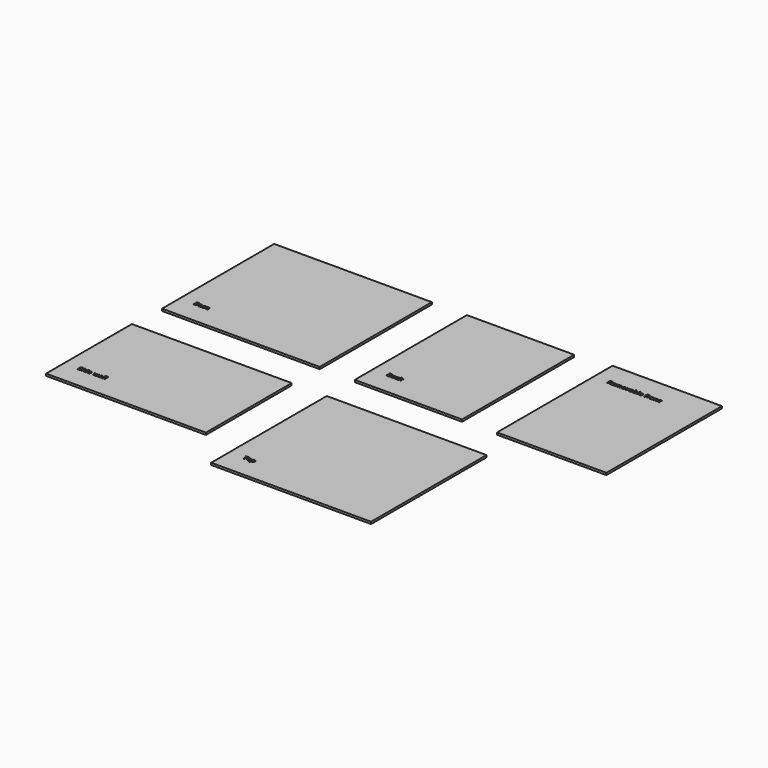
from build123d import *

# Parameters (mm, degrees)
F0_W     = 450
F0_H     = 400
F1_DEPTH = 6
F0_W_2   = 306
F2_DEPTH = 6
F0_W_3   = 456
F0_H_2   = 306
F0_W_4   = 2.7071983507
F0_H_3   = 9.9254470486
F0_H_4   = 13.8143815104
F3_DEPTH = 6
F0_H_5   = 412
F4_DEPTH = 6
F0_W_5   = 312
F5_DEPTH = 6


with BuildPart() as f1:
    # F0 (on Top) → F1 (new body)
    with BuildSketch(Plane.XY):
        with Locations((-275, 250)):
            Rectangle(F0_W, F0_H)
        with BuildLine():
            Line((-438.1719704861, 110), (-440.0610438368, 110))
            Line((-440.0610438368, 110), (-440.5865755208, 111.3493381076))
            Line((-440.5865755208, 111.3493381076), (-440.657593316, 111.3493381076))
            add(Edge.make_bspline(
                [(-440.657593316, 111.3493381076), (-441.3393641493, 110.4886024306), (-442.0637456597, 110.1548187934)],
                knots=[0, 0, 0, 1, 1, 1], degree=2))
            add(Edge.make_bspline(
                [(-442.0637456597, 110.1548187934), (-442.7881271701, 109.8210351562), (-443.9499782986, 109.8210351562)],
                knots=[0, 0, 0, 1, 1, 1], degree=2))
            add(Edge.make_bspline(
                [(-443.9499782986, 109.8210351562), (-445.3788563368, 109.8210351562), (-446.1998220486, 110.6391601562)],
                knots=[0, 0, 0, 1, 1, 1], degree=2))
            add(Edge.make_bspline(
                [(-446.1998220486, 110.6391601562), (-447.0207877604, 111.4572851562), (-447.0207877604, 112.965703125)],
                knots=[0, 0, 0, 1, 1, 1], degree=2))
            add(Edge.make_bspline(
                [(-447.0207877604, 112.965703125), (-447.0207877604, 114.5451388889), (-445.9157508681, 115.2950868056)],
                knots=[0, 0, 0, 1, 1, 1], degree=2))
            add(Edge.make_bspline(
                [(-445.9157508681, 115.2950868056), (-444.8107139757, 116.0450347222), (-442.5835959201, 116.1245746528)],
                knots=[0, 0, 0, 1, 1, 1], degree=2))
            Line((-442.5835959201, 116.1245746528), (-440.8592838542, 116.1785481771))
            Line((-440.8592838542, 116.1785481771), (-440.8592838542, 116.6131770833))
            add(Edge.make_bspline(
                [(-440.8592838542, 116.6131770833), (-440.8592838542, 118.1215950521), (-442.4046310764, 118.1215950521)],
                knots=[0, 0, 0, 1, 1, 1], degree=2))
            add(Edge.make_bspline(
                [(-442.4046310764, 118.1215950521), (-443.5948893229, 118.1215950521), (-445.2027322049, 117.4028949653)],
                knots=[0, 0, 0, 1, 1, 1], degree=2))
            Line((-445.2027322049, 117.4028949653), (-446.0975564236, 119.2323133681))
            add(Edge.make_bspline(
                [(-446.0975564236, 119.2323133681), (-444.3846072049, 120.1299782986), (-442.2995247396, 120.1299782986)],
                knots=[0, 0, 0, 1, 1, 1], degree=2))
            add(Edge.make_bspline(
                [(-442.2995247396, 120.1299782986), (-440.3025043403, 120.1299782986), (-439.2372374132, 119.2593001302)],
                knots=[0, 0, 0, 1, 1, 1], degree=2))
            add(Edge.make_bspline(
                [(-439.2372374132, 119.2593001302), (-438.1719704861, 118.3886219618), (-438.1719704861, 116.6131770833)],
                knots=[0, 0, 0, 1, 1, 1], degree=2))
            Line((-438.1719704861, 116.6131770833), (-438.1719704861, 110))
        make_face(mode=Mode.SUBTRACT)
        with BuildLine():
            add(Edge.make_bspline(
                [(-428.7152408854, 114.2170366753), (-428.4567361111, 113.6844032118), (-428.4567361111, 112.9486588542)],
                knots=[0, 0, 0, 1, 1, 1], degree=2))
            add(Edge.make_bspline(
                [(-428.4567361111, 112.9486588542), (-428.4567361111, 111.4203559028), (-429.5177419705, 110.6206955295)],
                knots=[0, 0, 0, 1, 1, 1], degree=2))
            add(Edge.make_bspline(
                [(-429.5177419705, 110.6206955295), (-430.5787478299, 109.8210351562), (-432.6922374132, 109.8210351562)],
                knots=[0, 0, 0, 1, 1, 1], degree=2))
            add(Edge.make_bspline(
                [(-432.6922374132, 109.8210351562), (-433.7745486111, 109.8210351562), (-434.5387000868, 109.9687521701)],
                knots=[0, 0, 0, 1, 1, 1], degree=2))
            add(Edge.make_bspline(
                [(-434.5387000868, 109.9687521701), (-435.3028515625, 110.116469184), (-435.967578125, 110.4005403646)],
                knots=[0, 0, 0, 1, 1, 1], degree=2))
            Line((-435.967578125, 110.4005403646), (-435.967578125, 112.6361805556))
            add(Edge.make_bspline(
                [(-435.967578125, 112.6361805556), (-435.2147894965, 112.2810915799), (-434.2688324653, 112.0410514323)],
                knots=[0, 0, 0, 1, 1, 1], degree=2))
            add(Edge.make_bspline(
                [(-434.2688324653, 112.0410514323), (-433.322875434, 111.8010112847), (-432.6041753472, 111.8010112847)],
                knots=[0, 0, 0, 1, 1, 1], degree=2))
            add(Edge.make_bspline(
                [(-432.6041753472, 111.8010112847), (-431.1298459201, 111.8010112847), (-431.1298459201, 112.6532248264)],
                knots=[0, 0, 0, 1, 1, 1], degree=2))
            add(Edge.make_bspline(
                [(-431.1298459201, 112.6532248264), (-431.1298459201, 112.9742252604), (-431.3258550347, 113.1744954427)],
                knots=[0, 0, 0, 1, 1, 1], degree=2))
            add(Edge.make_bspline(
                [(-431.3258550347, 113.1744954427), (-431.5218641493, 113.374765625), (-432.0005240885, 113.6275889757)],
                knots=[0, 0, 0, 1, 1, 1], degree=2))
            add(Edge.make_bspline(
                [(-432.0005240885, 113.6275889757), (-432.4791840278, 113.8804123264), (-433.2774240451, 114.2156163194)],
                knots=[0, 0, 0, 1, 1, 1], degree=2))
            add(Edge.make_bspline(
                [(-433.2774240451, 114.2156163194), (-434.4222309028, 114.6956966146), (-434.9605457899, 115.1047591146)],
                knots=[0, 0, 0, 1, 1, 1], degree=2))
            add(Edge.make_bspline(
                [(-434.9605457899, 115.1047591146), (-435.4988606771, 115.5138216146), (-435.7417415365, 116.0421940104)],
                knots=[0, 0, 0, 1, 1, 1], degree=2))
            add(Edge.make_bspline(
                [(-435.7417415365, 116.0421940104), (-435.9846223958, 116.5705664062), (-435.9846223958, 117.3403993056)],
                knots=[0, 0, 0, 1, 1, 1], degree=2))
            add(Edge.make_bspline(
                [(-435.9846223958, 117.3403993056), (-435.9846223958, 118.6641710069), (-434.9605457899, 119.3871321615)],
                knots=[0, 0, 0, 1, 1, 1], degree=2))
            add(Edge.make_bspline(
                [(-434.9605457899, 119.3871321615), (-433.936469184, 120.110093316), (-432.0530772569, 120.110093316)],
                knots=[0, 0, 0, 1, 1, 1], degree=2))
            add(Edge.make_bspline(
                [(-432.0530772569, 120.110093316), (-430.2605881076, 120.110093316), (-428.5646831597, 119.3288975694)],
                knots=[0, 0, 0, 1, 1, 1], degree=2))
            Line((-428.5646831597, 119.3288975694), (-429.3799674479, 117.377328559))
            add(Edge.make_bspline(
                [(-429.3799674479, 117.377328559), (-430.1270746528, 117.6954882812), (-430.7747569444, 117.9000195312)],
                knots=[0, 0, 0, 1, 1, 1], degree=2))
            add(Edge.make_bspline(
                [(-430.7747569444, 117.9000195312), (-431.4224392361, 118.1045507812), (-432.0985286458, 118.1045507812)],
                knots=[0, 0, 0, 1, 1, 1], degree=2))
            add(Edge.make_bspline(
                [(-432.0985286458, 118.1045507812), (-433.2973090278, 118.1045507812), (-433.2973090278, 117.4568684896)],
                knots=[0, 0, 0, 1, 1, 1], degree=2))
            add(Edge.make_bspline(
                [(-433.2973090278, 117.4568684896), (-433.2973090278, 117.0932573785), (-432.9109722222, 116.8262304687)],
                knots=[0, 0, 0, 1, 1, 1], degree=2))
            add(Edge.make_bspline(
                [(-432.9109722222, 116.8262304687), (-432.5246354167, 116.559203559), (-431.2179079861, 116.0365125868)],
                knots=[0, 0, 0, 1, 1, 1], degree=2))
            add(Edge.make_bspline(
                [(-431.2179079861, 116.0365125868), (-430.0560568576, 115.5649544271), (-429.5149012587, 115.157312283)],
                knots=[0, 0, 0, 1, 1, 1], degree=2))
            add(Edge.make_bspline(
                [(-429.5149012587, 115.157312283), (-428.9737456597, 114.7496701389), (-428.7152408854, 114.2170366753)],
                knots=[0, 0, 0, 1, 1, 1], degree=2))
        make_face(mode=Mode.SUBTRACT)
        with BuildLine():
            add(Edge.make_bspline(
                [(-419.8834678819, 109.9943185764), (-420.6902300347, 109.8210351562), (-421.854921875, 109.8210351562)],
                knots=[0, 0, 0, 1, 1, 1], degree=2))
            add(Edge.make_bspline(
                [(-421.854921875, 109.8210351562), (-424.2496419271, 109.8210351562), (-425.5989800347, 111.1448068576)],
                knots=[0, 0, 0, 1, 1, 1], degree=2))
            add(Edge.make_bspline(
                [(-425.5989800347, 111.1448068576), (-426.9483181424, 112.468578559), (-426.9483181424, 114.8917057292)],
                knots=[0, 0, 0, 1, 1, 1], degree=2))
            add(Edge.make_bspline(
                [(-426.9483181424, 114.8917057292), (-426.9483181424, 117.3858506944), (-425.7012456597, 118.7479720052)],
                knots=[0, 0, 0, 1, 1, 1], degree=2))
            add(Edge.make_bspline(
                [(-425.7012456597, 118.7479720052), (-424.4541731771, 120.110093316), (-422.2526215278, 120.110093316)],
                knots=[0, 0, 0, 1, 1, 1], degree=2))
            add(Edge.make_bspline(
                [(-422.2526215278, 120.110093316), (-420.1504947917, 120.110093316), (-418.9787011719, 118.9127332899)],
                knots=[0, 0, 0, 1, 1, 1], degree=2))
            add(Edge.make_bspline(
                [(-418.9787011719, 118.9127332899), (-417.8069075521, 117.7153732639), (-417.8069075521, 115.6018836806)],
                knots=[0, 0, 0, 1, 1, 1], degree=2))
            Line((-417.8069075521, 115.6018836806), (-417.8069075521, 114.2866341146))
            Line((-417.8069075521, 114.2866341146), (-424.20703125, 114.2866341146))
            add(Edge.make_bspline(
                [(-424.20703125, 114.2866341146), (-424.1615798611, 113.1333051215), (-423.5224197049, 112.4856228299)],
                knots=[0, 0, 0, 1, 1, 1], degree=2))
            add(Edge.make_bspline(
                [(-423.5224197049, 112.4856228299), (-422.8832595486, 111.8379405382), (-421.7299305556, 111.8379405382)],
                knots=[0, 0, 0, 1, 1, 1], degree=2))
            add(Edge.make_bspline(
                [(-421.7299305556, 111.8379405382), (-420.832265625, 111.8379405382), (-420.0340256076, 112.0240071615)],
                knots=[0, 0, 0, 1, 1, 1], degree=2))
            add(Edge.make_bspline(
                [(-420.0340256076, 112.0240071615), (-419.2357855903, 112.2100737847), (-418.3665277778, 112.6191362847)],
                knots=[0, 0, 0, 1, 1, 1], degree=2))
            Line((-418.3665277778, 112.6191362847), (-418.3665277778, 110.5226909722))
            add(Edge.make_bspline(
                [(-418.3665277778, 110.5226909722), (-419.0767057292, 110.1676019965), (-419.8834678819, 109.9943185764)],
                knots=[0, 0, 0, 1, 1, 1], degree=2))
        make_face(mode=Mode.SUBTRACT)
        with BuildLine():
            Line((-458.3665907118, 110), (-458.3665907118, 122.9792122396))
            Line((-458.3665907118, 122.9792122396), (-454.3270985243, 122.9792122396))
            add(Edge.make_bspline(
                [(-454.3270985243, 122.9792122396), (-451.5659266493, 122.9792122396), (-450.3188541667, 122.1937554253)],
                knots=[0, 0, 0, 1, 1, 1], degree=2))
            add(Edge.make_bspline(
                [(-450.3188541667, 122.1937554253), (-449.071781684, 121.4082986111), (-449.071781684, 119.6953493924)],
                knots=[0, 0, 0, 1, 1, 1], degree=2))
            add(Edge.make_bspline(
                [(-449.071781684, 119.6953493924), (-449.071781684, 118.5306575521), (-449.6171983507, 117.7849707031)],
                knots=[0, 0, 0, 1, 1, 1], degree=2))
            add(Edge.make_bspline(
                [(-449.6171983507, 117.7849707031), (-450.1626150174, 117.0392838542), (-451.0688020833, 116.8887261285)],
                knots=[0, 0, 0, 1, 1, 1], degree=2))
            Line((-451.0688020833, 116.8887261285), (-451.0688020833, 116.8006640625))
            add(Edge.make_bspline(
                [(-451.0688020833, 116.8006640625), (-449.8359331597, 116.5251150174), (-449.2890961372, 115.770906033)],
                knots=[0, 0, 0, 1, 1, 1], degree=2))
            add(Edge.make_bspline(
                [(-449.2890961372, 115.770906033), (-448.7422591146, 115.0166970486), (-448.7422591146, 113.7639431424)],
                knots=[0, 0, 0, 1, 1, 1], degree=2))
            add(Edge.make_bspline(
                [(-448.7422591146, 113.7639431424), (-448.7422591146, 111.9884982639), (-450.0262608507, 110.9942491319)],
                knots=[0, 0, 0, 1, 1, 1], degree=2))
            add(Edge.make_bspline(
                [(-450.0262608507, 110.9942491319), (-451.3102625868, 110), (-453.5118142361, 110)],
                knots=[0, 0, 0, 1, 1, 1], degree=2))
            Line((-453.5118142361, 110), (-458.3665907118, 110))
        make_face(mode=Mode.SUBTRACT)
    extrude(amount=F1_DEPTH)


with BuildPart() as f2:
    # F0 (on Top) → F2 (new body)
    with BuildSketch(Plane.XY):
        with Locations((203, 250)):
            Rectangle(F0_W_2, F0_H)
        with BuildLine():
            Line((111.8281674137, 110), (109.9390821287, 110))
            Line((109.9390821287, 110), (109.4135471246, 111.3493466322))
            Line((109.4135471246, 111.3493466322), (109.3425288808, 111.3493466322))
            add(Edge.make_bspline(
                [(109.3425288808, 111.3493466322), (108.6607537403, 110.4886055173), (107.9363676536, 110.1548197715)],
                knots=[0, 0, 0, 1, 1, 1], degree=2))
            add(Edge.make_bspline(
                [(107.9363676536, 110.1548197715), (107.2119815668, 109.8210340256), (106.0501230983, 109.8210340256)],
                knots=[0, 0, 0, 1, 1, 1], degree=2))
            add(Edge.make_bspline(
                [(106.0501230983, 109.8210340256), (104.6212360331, 109.8210340256), (103.8002651348, 110.6391641942)],
                knots=[0, 0, 0, 1, 1, 1], degree=2))
            add(Edge.make_bspline(
                [(103.8002651348, 110.6391641942), (102.9792942365, 111.4572943627), (102.9792942365, 112.965721861)],
                knots=[0, 0, 0, 1, 1, 1], degree=2))
            add(Edge.make_bspline(
                [(102.9792942365, 112.965721861), (102.9792942365, 114.5451676031), (104.08433811, 115.2951202576)],
                knots=[0, 0, 0, 1, 1, 1], degree=2))
            add(Edge.make_bspline(
                [(104.08433811, 115.2951202576), (105.1893819835, 116.0450729121), (107.416514109, 116.1246133451)],
                knots=[0, 0, 0, 1, 1, 1], degree=2))
            Line((107.416514109, 116.1246133451), (109.1408370684, 116.1785872104))
            Line((109.1408370684, 116.1785872104), (109.1408370684, 116.6132188624))
            add(Edge.make_bspline(
                [(109.1408370684, 116.6132188624), (109.1408370684, 118.1216463607), (107.5954800833, 118.1216463607)],
                knots=[0, 0, 0, 1, 1, 1], degree=2))
            add(Edge.make_bspline(
                [(107.5954800833, 118.1216463607), (106.4052143173, 118.1216463607), (104.7973612777, 117.4029417335)],
                knots=[0, 0, 0, 1, 1, 1], degree=2))
            Line((104.7973612777, 117.4029417335), (103.9025314058, 119.2323716937))
            add(Edge.make_bspline(
                [(103.9025314058, 119.2323716937), (105.6154914462, 120.1300422953), (107.7005870841, 120.1300422953)],
                knots=[0, 0, 0, 1, 1, 1], degree=2))
            add(Edge.make_bspline(
                [(107.7005870841, 120.1300422953), (109.6976200997, 120.1300422953), (110.7628937567, 119.2593586263)],
                knots=[0, 0, 0, 1, 1, 1], degree=2))
            add(Edge.make_bspline(
                [(110.7628937567, 119.2593586263), (111.8281674137, 118.3886749574), (111.8281674137, 116.6132188624)],
                knots=[0, 0, 0, 1, 1, 1], degree=2))
            Line((111.8281674137, 116.6132188624), (111.8281674137, 110))
        make_face(mode=Mode.SUBTRACT)
        with BuildLine():
            add(Edge.make_bspline(
                [(120.3389937504, 109.9815352566), (119.6685815289, 109.8210340256), (118.648759548, 109.8210340256)],
                knots=[0, 0, 0, 1, 1, 1], degree=2))
            add(Edge.make_bspline(
                [(118.648759548, 109.8210340256), (114.0155293226, 109.8210340256), (114.0155293226, 114.9087810113)],
                knots=[0, 0, 0, 1, 1, 1], degree=2))
            add(Edge.make_bspline(
                [(114.0155293226, 114.9087810113), (114.0155293226, 117.4398712203), (115.2753929676, 118.7750142036)],
                knots=[0, 0, 0, 1, 1, 1], degree=2))
            add(Edge.make_bspline(
                [(115.2753929676, 118.7750142036), (116.5352566126, 120.110157187), (118.8873808472, 120.110157187)],
                knots=[0, 0, 0, 1, 1, 1], degree=2))
            add(Edge.make_bspline(
                [(118.8873808472, 120.110157187), (120.6088630768, 120.110157187), (121.9780948172, 119.4369042358)],
                knots=[0, 0, 0, 1, 1, 1], degree=2))
            Line((121.9780948172, 119.4369042358), (121.1770090272, 117.3404456789))
            add(Edge.make_bspline(
                [(121.1770090272, 117.3404456789), (120.537844833, 117.5989520864), (119.988163626, 117.763714412)],
                knots=[0, 0, 0, 1, 1, 1], degree=2))
            add(Edge.make_bspline(
                [(119.988163626, 117.763714412), (119.438482419, 117.9284767376), (118.8873808472, 117.9284767376)],
                knots=[0, 0, 0, 1, 1, 1], degree=2))
            add(Edge.make_bspline(
                [(118.8873808472, 117.9284767376), (116.7738779117, 117.9284767376), (116.7738779117, 114.9258253898)],
                knots=[0, 0, 0, 1, 1, 1], degree=2))
            add(Edge.make_bspline(
                [(116.7738779117, 114.9258253898), (116.7738779117, 112.0140773941), (118.8873808472, 112.0140773941)],
                knots=[0, 0, 0, 1, 1, 1], degree=2))
            add(Edge.make_bspline(
                [(118.8873808472, 112.0140773941), (119.6685815289, 112.0140773941), (120.3347326558, 112.2228710309)],
                knots=[0, 0, 0, 1, 1, 1], degree=2))
            add(Edge.make_bspline(
                [(120.3347326558, 112.2228710309), (121.0008837826, 112.4316646676), (121.6656145445, 112.8776592387)],
                knots=[0, 0, 0, 1, 1, 1], degree=2))
            Line((121.6656145445, 112.8776592387), (121.6656145445, 110.5596237611))
            add(Edge.make_bspline(
                [(121.6656145445, 110.5596237611), (121.0094059718, 110.1420364876), (120.3389937504, 109.9815352566)],
                knots=[0, 0, 0, 1, 1, 1], degree=2))
        make_face(mode=Mode.SUBTRACT)
        with BuildLine():
            Line((91.6334196073, 110), (91.6334196073, 122.9792942365))
            Line((91.6334196073, 122.9792942365), (95.6729373146, 122.9792942365))
            add(Edge.make_bspline(
                [(95.6729373146, 122.9792942365), (98.4341266334, 122.9792942365), (99.6812069945, 122.1938324601)],
                knots=[0, 0, 0, 1, 1, 1], degree=2))
            add(Edge.make_bspline(
                [(99.6812069945, 122.1938324601), (100.9282873556, 121.4083706837), (100.9282873556, 119.6954106433)],
                knots=[0, 0, 0, 1, 1, 1], degree=2))
            add(Edge.make_bspline(
                [(100.9282873556, 119.6954106433), (100.9282873556, 118.530711445), (100.3828672432, 117.7850198851)],
                knots=[0, 0, 0, 1, 1, 1], degree=2))
            add(Edge.make_bspline(
                [(100.3828672432, 117.7850198851), (99.8374471309, 117.0393283252), (98.93125434, 116.8887696484)],
                knots=[0, 0, 0, 1, 1, 1], degree=2))
            Line((98.93125434, 116.8887696484), (98.93125434, 116.8007070261))
            add(Edge.make_bspline(
                [(98.93125434, 116.8007070261), (100.1641310523, 116.5251562401), (100.7109715296, 115.770942491)],
                knots=[0, 0, 0, 1, 1, 1], degree=2))
            add(Edge.make_bspline(
                [(100.7109715296, 115.770942491), (101.2578120068, 115.0167287419), (101.2578120068, 113.7639669213)],
                knots=[0, 0, 0, 1, 1, 1], degree=2))
            add(Edge.make_bspline(
                [(101.2578120068, 113.7639669213), (101.2578120068, 111.9885108263), (99.973802159, 110.9942554132)],
                knots=[0, 0, 0, 1, 1, 1], degree=2))
            add(Edge.make_bspline(
                [(99.973802159, 110.9942554132), (98.6897923111, 110), (96.4882267534, 110)],
                knots=[0, 0, 0, 1, 1, 1], degree=2))
            Line((96.4882267534, 110), (91.6334196073, 110))
        make_face(mode=Mode.SUBTRACT)
        Polygon((126.5317846096, 115.3973865286), (126.5687140963, 115.3973865286), (127.7476169434, 116.9058140269), (130.5258506407, 119.9255097532), (133.579635124, 119.9255097532), (129.6395429581, 115.6189634493), (133.821097153, 110), (130.6962944259, 110), (127.8385202954, 114.0224733287), (126.6738210972, 113.0907139701), (126.6738210972, 110), (123.9666056436, 110), (123.9666056436, 123.8144687835), (126.6738210972, 123.8144687835), (126.6738210972, 117.6529259516), align=None, mode=Mode.SUBTRACT)
    extrude(amount=F2_DEPTH)


with BuildPart() as f3:
    # F0 (on Top) → F3 (new body)
    with BuildSketch(Plane.XY):
        with Locations((-278, -203)):
            Rectangle(F0_W_3, F0_H_2)
        with BuildLine():
            add(Edge.make_bspline(
                [(-457.379860026, -290.2518196615), (-456.7051909722, -291.1253385417), (-456.7051909722, -292.3951367188)],
                knots=[0, 0, 0, 1, 1, 1], degree=2))
            add(Edge.make_bspline(
                [(-456.7051909722, -292.3951367188), (-456.7051909722, -294.1535373264), (-457.9707280816, -295.1662510851)],
                knots=[0, 0, 0, 1, 1, 1], degree=2))
            add(Edge.make_bspline(
                [(-457.9707280816, -295.1662510851), (-459.236265191, -296.1789648438), (-461.4889496528, -296.1789648438)],
                knots=[0, 0, 0, 1, 1, 1], degree=2))
            add(Edge.make_bspline(
                [(-461.4889496528, -296.1789648438), (-463.5683506944, -296.1789648438), (-465.1648307292, -295.3949283854)],
                knots=[0, 0, 0, 1, 1, 1], degree=2))
            Line((-465.1648307292, -295.3949283854), (-465.1648307292, -292.8382877604))
            add(Edge.make_bspline(
                [(-465.1648307292, -292.8382877604), (-463.852421875, -293.4263151042), (-462.9419737413, -293.6649348958)],
                knots=[0, 0, 0, 1, 1, 1], degree=2))
            add(Edge.make_bspline(
                [(-462.9419737413, -293.6649348958), (-462.0315256076, -293.9035546875), (-461.2758962674, -293.9035546875)],
                knots=[0, 0, 0, 1, 1, 1], degree=2))
            add(Edge.make_bspline(
                [(-461.2758962674, -293.9035546875), (-460.3725499132, -293.9035546875), (-459.8882085503, -293.5584082031)],
                knots=[0, 0, 0, 1, 1, 1], degree=2))
            add(Edge.make_bspline(
                [(-459.8882085503, -293.5584082031), (-459.4038671875, -293.2132617188), (-459.4038671875, -292.5286501736)],
                knots=[0, 0, 0, 1, 1, 1], degree=2))
            add(Edge.make_bspline(
                [(-459.4038671875, -292.5286501736), (-459.4038671875, -292.1479947917), (-459.6169205729, -291.8497200521)],
                knots=[0, 0, 0, 1, 1, 1], degree=2))
            add(Edge.make_bspline(
                [(-459.6169205729, -291.8497200521), (-459.8299739583, -291.5514453125), (-460.243297526, -291.2773166233)],
                knots=[0, 0, 0, 1, 1, 1], degree=2))
            add(Edge.make_bspline(
                [(-460.243297526, -291.2773166233), (-460.6566210937, -291.003187934), (-461.9264192708, -290.3981163194)],
                knots=[0, 0, 0, 1, 1, 1], degree=2))
            add(Edge.make_bspline(
                [(-461.9264192708, -290.3981163194), (-463.1138368056, -289.8384960938), (-463.7089659288, -289.3243272569)],
                knots=[0, 0, 0, 1, 1, 1], degree=2))
            add(Edge.make_bspline(
                [(-463.7089659288, -289.3243272569), (-464.3040950521, -288.8101584201), (-464.6591840278, -288.125546875)],
                knots=[0, 0, 0, 1, 1, 1], degree=2))
            add(Edge.make_bspline(
                [(-464.6591840278, -288.125546875), (-465.0142730035, -287.4409353299), (-465.0142730035, -286.5290668403)],
                knots=[0, 0, 0, 1, 1, 1], degree=2))
            add(Edge.make_bspline(
                [(-465.0142730035, -286.5290668403), (-465.0142730035, -284.8047547743), (-463.8467404514, -283.8204481337)],
                knots=[0, 0, 0, 1, 1, 1], degree=2))
            add(Edge.make_bspline(
                [(-463.8467404514, -283.8204481337), (-462.6792078993, -282.8361414931), (-460.6196918403, -282.8361414931)],
                knots=[0, 0, 0, 1, 1, 1], degree=2))
            add(Edge.make_bspline(
                [(-460.6196918403, -282.8361414931), (-459.6083984375, -282.8361414931), (-458.6894281684, -283.0747612847)],
                knots=[0, 0, 0, 1, 1, 1], degree=2))
            add(Edge.make_bspline(
                [(-458.6894281684, -283.0747612847), (-457.7704578993, -283.3133810764), (-456.7676866319, -283.7480099826)],
                knots=[0, 0, 0, 1, 1, 1], degree=2))
            Line((-456.7676866319, -283.7480099826), (-457.6539887153, -285.889906684))
            add(Edge.make_bspline(
                [(-457.6539887153, -285.889906684), (-458.6936892361, -285.4637999132), (-459.3726193576, -285.2947775608)],
                knots=[0, 0, 0, 1, 1, 1], degree=2))
            add(Edge.make_bspline(
                [(-459.3726193576, -285.2947775608), (-460.0515494792, -285.1257552083), (-460.7077539062, -285.1257552083)],
                knots=[0, 0, 0, 1, 1, 1], degree=2))
            add(Edge.make_bspline(
                [(-460.7077539062, -285.1257552083), (-461.4889496528, -285.1257552083), (-461.9065342882, -285.4893663194)],
                knots=[0, 0, 0, 1, 1, 1], degree=2))
            add(Edge.make_bspline(
                [(-461.9065342882, -285.4893663194), (-462.3241189236, -285.8529774306), (-462.3241189236, -286.4381640625)],
                knots=[0, 0, 0, 1, 1, 1], degree=2))
            add(Edge.make_bspline(
                [(-462.3241189236, -286.4381640625), (-462.3241189236, -286.8017751736), (-462.1550965712, -287.073063151)],
                knots=[0, 0, 0, 1, 1, 1], degree=2))
            add(Edge.make_bspline(
                [(-462.1550965712, -287.073063151), (-461.9860742187, -287.3443511285), (-461.6182020399, -287.5971744792)],
                knots=[0, 0, 0, 1, 1, 1], degree=2))
            add(Edge.make_bspline(
                [(-461.6182020399, -287.5971744792), (-461.2503298611, -287.8499978299), (-459.8754253472, -288.5062022569)],
                knots=[0, 0, 0, 1, 1, 1], degree=2))
            add(Edge.make_bspline(
                [(-459.8754253472, -288.5062022569), (-458.0545290799, -289.3783007813), (-457.379860026, -290.2518196615)],
                knots=[0, 0, 0, 1, 1, 1], degree=2))
        make_face(mode=Mode.SUBTRACT)
        with Locations((-453.2125358073, -291.0372764757)):
            Rectangle(F0_W_4, F0_H_3, mode=Mode.SUBTRACT)
        with BuildLine():
            add(Edge.make_bspline(
                [(-443.0612521701, -294.7131575521), (-443.9844835069, -296.1789648438), (-445.8763975694, -296.1789648438)],
                knots=[0, 0, 0, 1, 1, 1], degree=2))
            add(Edge.make_bspline(
                [(-445.8763975694, -296.1789648438), (-447.6234353299, -296.1789648438), (-448.6219455295, -294.8196842448)],
                knots=[0, 0, 0, 1, 1, 1], degree=2))
            add(Edge.make_bspline(
                [(-448.6219455295, -294.8196842448), (-449.6204557292, -293.4604036458), (-449.6204557292, -291.0543207465)],
                knots=[0, 0, 0, 1, 1, 1], degree=2))
            add(Edge.make_bspline(
                [(-449.6204557292, -291.0543207465), (-449.6204557292, -288.6141493056), (-448.6049012587, -287.2520279948)],
                knots=[0, 0, 0, 1, 1, 1], degree=2))
            add(Edge.make_bspline(
                [(-448.6049012587, -287.2520279948), (-447.5893467882, -285.889906684), (-445.8053797743, -285.889906684)],
                knots=[0, 0, 0, 1, 1, 1], degree=2))
            add(Edge.make_bspline(
                [(-445.8053797743, -285.889906684), (-443.9305099826, -285.889906684), (-442.9447829861, -287.3443511285)],
                knots=[0, 0, 0, 1, 1, 1], degree=2))
            Line((-442.9447829861, -287.3443511285), (-442.8567209201, -287.3443511285))
            add(Edge.make_bspline(
                [(-442.8567209201, -287.3443511285), (-443.0612521701, -286.2336328125), (-443.0612521701, -285.364375)],
                knots=[0, 0, 0, 1, 1, 1], degree=2))
            Line((-443.0612521701, -285.364375), (-443.0612521701, -282.1856184896))
            Line((-443.0612521701, -282.1856184896), (-440.345531684, -282.1856184896))
            Line((-440.345531684, -282.1856184896), (-440.345531684, -296))
            Line((-440.345531684, -296), (-442.4220920139, -296))
            Line((-442.4220920139, -296), (-442.9447829861, -294.7131575521))
            Line((-442.9447829861, -294.7131575521), (-443.0612521701, -294.7131575521))
        make_face(mode=Mode.SUBTRACT)
        with BuildLine():
            add(Edge.make_bspline(
                [(-431.0507226562, -296.0056814236), (-431.857484809, -296.1789648438), (-433.0221766493, -296.1789648438)],
                knots=[0, 0, 0, 1, 1, 1], degree=2))
            add(Edge.make_bspline(
                [(-433.0221766493, -296.1789648438), (-435.4168967014, -296.1789648438), (-436.766234809, -294.8551931424)],
                knots=[0, 0, 0, 1, 1, 1], degree=2))
            add(Edge.make_bspline(
                [(-436.766234809, -294.8551931424), (-438.1155729167, -293.531421441), (-438.1155729167, -291.1082942708)],
                knots=[0, 0, 0, 1, 1, 1], degree=2))
            add(Edge.make_bspline(
                [(-438.1155729167, -291.1082942708), (-438.1155729167, -288.6141493056), (-436.868500434, -287.2520279948)],
                knots=[0, 0, 0, 1, 1, 1], degree=2))
            add(Edge.make_bspline(
                [(-436.868500434, -287.2520279948), (-435.6214279514, -285.889906684), (-433.4198763021, -285.889906684)],
                knots=[0, 0, 0, 1, 1, 1], degree=2))
            add(Edge.make_bspline(
                [(-433.4198763021, -285.889906684), (-431.317749566, -285.889906684), (-430.1459559462, -287.0872667101)],
                knots=[0, 0, 0, 1, 1, 1], degree=2))
            add(Edge.make_bspline(
                [(-430.1459559462, -287.0872667101), (-428.9741623264, -288.2846267361), (-428.9741623264, -290.3981163194)],
                knots=[0, 0, 0, 1, 1, 1], degree=2))
            Line((-428.9741623264, -290.3981163194), (-428.9741623264, -291.7133658854))
            Line((-428.9741623264, -291.7133658854), (-435.3742860243, -291.7133658854))
            add(Edge.make_bspline(
                [(-435.3742860243, -291.7133658854), (-435.3288346354, -292.8666948785), (-434.6896744792, -293.5143771701)],
                knots=[0, 0, 0, 1, 1, 1], degree=2))
            add(Edge.make_bspline(
                [(-434.6896744792, -293.5143771701), (-434.0505143229, -294.1620594618), (-432.8971853299, -294.1620594618)],
                knots=[0, 0, 0, 1, 1, 1], degree=2))
            add(Edge.make_bspline(
                [(-432.8971853299, -294.1620594618), (-431.9995203993, -294.1620594618), (-431.2012803819, -293.9759928385)],
                knots=[0, 0, 0, 1, 1, 1], degree=2))
            add(Edge.make_bspline(
                [(-431.2012803819, -293.9759928385), (-430.4030403646, -293.7899262153), (-429.5337825521, -293.3808637153)],
                knots=[0, 0, 0, 1, 1, 1], degree=2))
            Line((-429.5337825521, -293.3808637153), (-429.5337825521, -295.4773090278))
            add(Edge.make_bspline(
                [(-429.5337825521, -295.4773090278), (-430.2439605035, -295.8323980035), (-431.0507226562, -296.0056814236)],
                knots=[0, 0, 0, 1, 1, 1], degree=2))
        make_face(mode=Mode.SUBTRACT)
        with BuildLine():
            Line((-410.9441644965, -296), (-413.8899826389, -296))
            Line((-413.8899826389, -296), (-414.6541341146, -292.5286501736))
            Line((-414.6541341146, -292.5286501736), (-415.6824717882, -288.1425911458))
            Line((-415.6824717882, -288.1425911458), (-415.7449674479, -288.1425911458))
            Line((-415.7449674479, -288.1425911458), (-417.5573415799, -296))
            Line((-417.5573415799, -296), (-420.4690711806, -296))
            Line((-420.4690711806, -296), (-423.2898980035, -286.0745529514))
            Line((-423.2898980035, -286.0745529514), (-420.5912217882, -286.0745529514))
            Line((-420.5912217882, -286.0745529514), (-419.4464149306, -290.4691341146))
            add(Edge.make_bspline(
                [(-419.4464149306, -290.4691341146), (-419.1708658854, -291.6508702257), (-418.8867947049, -293.7274305556)],
                knots=[0, 0, 0, 1, 1, 1], degree=2))
            Line((-418.8867947049, -293.7274305556), (-418.8356618924, -293.7274305556))
            add(Edge.make_bspline(
                [(-418.8356618924, -293.7274305556), (-418.7987326389, -293.0513411458), (-418.5231835937, -291.588374566)],
                knots=[0, 0, 0, 1, 1, 1], degree=2))
            Line((-418.5231835937, -291.588374566), (-418.3811480035, -290.8327452257))
            Line((-418.3811480035, -290.8327452257), (-417.1568012153, -286.0745529514))
            Line((-417.1568012153, -286.0745529514), (-414.1740538194, -286.0745529514))
            Line((-414.1740538194, -286.0745529514), (-413.012202691, -290.8327452257))
            add(Edge.make_bspline(
                [(-413.012202691, -290.8327452257), (-412.9752734375, -291.0287543403), (-412.8999945747, -291.4108300781)],
                knots=[0, 0, 0, 1, 1, 1], degree=2))
            add(Edge.make_bspline(
                [(-412.8999945747, -291.4108300781), (-412.8247157118, -291.792905816), (-412.7536979167, -292.2232736545)],
                knots=[0, 0, 0, 1, 1, 1], degree=2))
            add(Edge.make_bspline(
                [(-412.7536979167, -292.2232736545), (-412.6826801215, -292.6536414931), (-412.6244455295, -293.0655447049)],
                knots=[0, 0, 0, 1, 1, 1], degree=2))
            add(Edge.make_bspline(
                [(-412.6244455295, -293.0655447049), (-412.5662109375, -293.4774479167), (-412.5576888021, -293.7274305556)],
                knots=[0, 0, 0, 1, 1, 1], degree=2))
            Line((-412.5576888021, -293.7274305556), (-412.5065559896, -293.7274305556))
            add(Edge.make_bspline(
                [(-412.5065559896, -293.7274305556), (-412.4241753472, -293.0882703993), (-412.2210644531, -291.9747113715)],
                knots=[0, 0, 0, 1, 1, 1], degree=2))
            add(Edge.make_bspline(
                [(-412.2210644531, -291.9747113715), (-412.017953559, -290.8611523438), (-411.9270507812, -290.4691341146)],
                knots=[0, 0, 0, 1, 1, 1], degree=2))
            Line((-411.9270507812, -290.4691341146), (-410.7396332465, -286.0745529514))
            Line((-410.7396332465, -286.0745529514), (-408.0835677083, -286.0745529514))
            Line((-408.0835677083, -286.0745529514), (-410.9441644965, -296))
        make_face(mode=Mode.SUBTRACT)
        with BuildLine():
            Line((-398.2944748264, -296), (-400.1835481771, -296))
            Line((-400.1835481771, -296), (-400.7090798611, -294.6506618924))
            Line((-400.7090798611, -294.6506618924), (-400.7800976562, -294.6506618924))
            add(Edge.make_bspline(
                [(-400.7800976562, -294.6506618924), (-401.4618684896, -295.5113975694), (-402.18625, -295.8451812066)],
                knots=[0, 0, 0, 1, 1, 1], degree=2))
            add(Edge.make_bspline(
                [(-402.18625, -295.8451812066), (-402.9106315104, -296.1789648438), (-404.0724826389, -296.1789648438)],
                knots=[0, 0, 0, 1, 1, 1], degree=2))
            add(Edge.make_bspline(
                [(-404.0724826389, -296.1789648438), (-405.5013606771, -296.1789648438), (-406.3223263889, -295.3608398438)],
                knots=[0, 0, 0, 1, 1, 1], degree=2))
            add(Edge.make_bspline(
                [(-406.3223263889, -295.3608398438), (-407.1432921007, -294.5427148438), (-407.1432921007, -293.034296875)],
                knots=[0, 0, 0, 1, 1, 1], degree=2))
            add(Edge.make_bspline(
                [(-407.1432921007, -293.034296875), (-407.1432921007, -291.4548611111), (-406.0382552083, -290.7049131944)],
                knots=[0, 0, 0, 1, 1, 1], degree=2))
            add(Edge.make_bspline(
                [(-406.0382552083, -290.7049131944), (-404.933218316, -289.9549652778), (-402.7061002604, -289.8754253472)],
                knots=[0, 0, 0, 1, 1, 1], degree=2))
            Line((-402.7061002604, -289.8754253472), (-400.9817881944, -289.8214518229))
            Line((-400.9817881944, -289.8214518229), (-400.9817881944, -289.3868229167))
            add(Edge.make_bspline(
                [(-400.9817881944, -289.3868229167), (-400.9817881944, -287.8784049479), (-402.5271354167, -287.8784049479)],
                knots=[0, 0, 0, 1, 1, 1], degree=2))
            add(Edge.make_bspline(
                [(-402.5271354167, -287.8784049479), (-403.7173936632, -287.8784049479), (-405.3252365451, -288.5971050347)],
                knots=[0, 0, 0, 1, 1, 1], degree=2))
            Line((-405.3252365451, -288.5971050347), (-406.2200607639, -286.7676866319))
            add(Edge.make_bspline(
                [(-406.2200607639, -286.7676866319), (-404.5071115451, -285.8700217014), (-402.4220290799, -285.8700217014)],
                knots=[0, 0, 0, 1, 1, 1], degree=2))
            add(Edge.make_bspline(
                [(-402.4220290799, -285.8700217014), (-400.4250086806, -285.8700217014), (-399.3597417535, -286.7406998698)],
                knots=[0, 0, 0, 1, 1, 1], degree=2))
            add(Edge.make_bspline(
                [(-399.3597417535, -286.7406998698), (-398.2944748264, -287.6113780382), (-398.2944748264, -289.3868229167)],
                knots=[0, 0, 0, 1, 1, 1], degree=2))
            Line((-398.2944748264, -289.3868229167), (-398.2944748264, -296))
        make_face(mode=Mode.SUBTRACT)
        with Locations((-394.151296658, -289.0928092448)):
            Rectangle(F0_W_4, F0_H_4, mode=Mode.SUBTRACT)
        with Locations((-388.6033865017, -289.0928092448)):
            Rectangle(F0_W_4, F0_H_4, mode=Mode.SUBTRACT)
        with BuildLine():
            add(Edge.make_bspline(
                [(-453.2082747396, -284.8416840278), (-454.6826041667, -284.8416840278), (-454.6826041667, -283.509390191)],
                knots=[0, 0, 0, 1, 1, 1], degree=2))
            add(Edge.make_bspline(
                [(-454.6826041667, -283.509390191), (-454.6826041667, -282.1856184896), (-453.2082747396, -282.1856184896)],
                knots=[0, 0, 0, 1, 1, 1], degree=2))
            add(Edge.make_bspline(
                [(-453.2082747396, -282.1856184896), (-451.7339453125, -282.1856184896), (-451.7339453125, -283.509390191)],
                knots=[0, 0, 0, 1, 1, 1], degree=2))
            add(Edge.make_bspline(
                [(-451.7339453125, -283.509390191), (-451.7339453125, -284.1400282118), (-452.1018174913, -284.4908561198)],
                knots=[0, 0, 0, 1, 1, 1], degree=2))
            add(Edge.make_bspline(
                [(-452.1018174913, -284.4908561198), (-452.4696896701, -284.8416840278), (-453.2082747396, -284.8416840278)],
                knots=[0, 0, 0, 1, 1, 1], degree=2))
        make_face(mode=Mode.SUBTRACT)
    extrude(amount=F3_DEPTH)


with BuildPart() as f4:
    # F0 (on Top) → F4 (new body)
    with BuildSketch(Plane.XY):
        with Locations((278, -256)):
            Rectangle(F0_W_3, F0_H_5)
        with BuildLine():
            add(Edge.make_bspline(
                [(110.3821072049, -394.2945692274), (110.9672938368, -395.4578407118), (110.9672938368, -397.0202322049)],
                knots=[0, 0, 0, 1, 1, 1], degree=2))
            add(Edge.make_bspline(
                [(110.9672938368, -397.0202322049), (110.9672938368, -399.443359375), (109.6889735243, -400.8111621094)],
                knots=[0, 0, 0, 1, 1, 1], degree=2))
            add(Edge.make_bspline(
                [(109.6889735243, -400.8111621094), (108.4106532118, -402.1789648437), (106.1295616319, -402.1789648437)],
                knots=[0, 0, 0, 1, 1, 1], degree=2))
            add(Edge.make_bspline(
                [(106.1295616319, -402.1789648437), (104.7006835938, -402.1789648437), (103.6084299045, -401.5525878906)],
                knots=[0, 0, 0, 1, 1, 1], degree=2))
            add(Edge.make_bspline(
                [(103.6084299045, -401.5525878906), (102.5161762153, -400.9262109375), (101.9309895833, -399.7544173177)],
                knots=[0, 0, 0, 1, 1, 1], degree=2))
            add(Edge.make_bspline(
                [(101.9309895833, -399.7544173177), (101.3458029514, -398.5826236979), (101.3458029514, -397.0202322049)],
                knots=[0, 0, 0, 1, 1, 1], degree=2))
            add(Edge.make_bspline(
                [(101.3458029514, -397.0202322049), (101.3458029514, -394.5885828993), (102.6141807726, -393.2392447917)],
                knots=[0, 0, 0, 1, 1, 1], degree=2))
            add(Edge.make_bspline(
                [(102.6141807726, -393.2392447917), (103.8825585938, -391.889906684), (106.1835351563, -391.889906684)],
                knots=[0, 0, 0, 1, 1, 1], degree=2))
            add(Edge.make_bspline(
                [(106.1835351563, -391.889906684), (107.6124131944, -391.889906684), (108.7046668837, -392.5106022135)],
                knots=[0, 0, 0, 1, 1, 1], degree=2))
            add(Edge.make_bspline(
                [(108.7046668837, -392.5106022135), (109.7969205729, -393.1312977431), (110.3821072049, -394.2945692274)],
                knots=[0, 0, 0, 1, 1, 1], degree=2))
        make_face(mode=Mode.SUBTRACT)
        Polygon((96.6415842014, -391.3104014757), (96.6415842014, -402), (93.8889344618, -402), (93.8889344618, -391.3104014757), (90.3636111111, -391.3104014757), (90.3636111111, -389.0207877604), (100.1640668403, -389.0207877604), (100.1640668403, -391.3104014757), align=None, mode=Mode.SUBTRACT)
        with BuildLine():
            add(Edge.make_bspline(
                [(120.6796875, -401.5653710937), (119.8189518229, -402.1789648437), (118.6571006944, -402.1789648437)],
                knots=[0, 0, 0, 1, 1, 1], degree=2))
            add(Edge.make_bspline(
                [(118.6571006944, -402.1789648437), (116.9072222222, -402.1789648437), (115.9129730903, -400.9091666667)],
                knots=[0, 0, 0, 1, 1, 1], degree=2))
            Line((115.9129730903, -400.9091666667), (115.7709375, -400.9091666667))
            add(Edge.make_bspline(
                [(115.7709375, -400.9091666667), (115.9129730903, -402.1505577257), (115.9129730903, -402.3465668403)],
                knots=[0, 0, 0, 1, 1, 1], degree=2))
            Line((115.9129730903, -402.3465668403), (115.9129730903, -406.3690147569))
            Line((115.9129730903, -406.3690147569), (113.2057747396, -406.3690147569))
            Line((113.2057747396, -406.3690147569), (113.2057747396, -392.0745529514))
            Line((113.2057747396, -392.0745529514), (115.4073263889, -392.0745529514))
            Line((115.4073263889, -392.0745529514), (115.7879817708, -393.3613953993))
            Line((115.7879817708, -393.3613953993), (115.9129730903, -393.3613953993))
            add(Edge.make_bspline(
                [(115.9129730903, -393.3613953993), (116.8646115451, -391.889906684), (118.7281184896, -391.889906684)],
                knots=[0, 0, 0, 1, 1, 1], degree=2))
            add(Edge.make_bspline(
                [(118.7281184896, -391.889906684), (120.4865190972, -391.889906684), (121.4807682292, -393.2477669271)],
                knots=[0, 0, 0, 1, 1, 1], degree=2))
            add(Edge.make_bspline(
                [(121.4807682292, -393.2477669271), (122.4750173611, -394.6056271701), (122.4750173611, -397.0202322049)],
                knots=[0, 0, 0, 1, 1, 1], degree=2))
            add(Edge.make_bspline(
                [(122.4750173611, -397.0202322049), (122.4750173611, -398.6081901042), (122.0077202691, -399.779983724)],
                knots=[0, 0, 0, 1, 1, 1], degree=2))
            add(Edge.make_bspline(
                [(122.0077202691, -399.779983724), (121.5404231771, -400.9517773437), (120.6796875, -401.5653710937)],
                knots=[0, 0, 0, 1, 1, 1], degree=2))
        make_face(mode=Mode.SUBTRACT)
    extrude(amount=F4_DEPTH)


with BuildPart() as f5:
    # F0 (on Top) → F5 (new body)
    with BuildSketch(Plane.XY):
        with Locations((612, 256)):
            Rectangle(F0_W_5, F0_H_5)
        with BuildLine():
            Line((501.8490256076, 393.8897677951), (500.3860590278, 393.8897677951))
            Line((500.3860590278, 393.8897677951), (500.3860590278, 388.91))
            Line((500.3860590278, 388.91), (497.6334092882, 388.91))
            Line((497.6334092882, 388.91), (497.6334092882, 401.8892122396))
            Line((497.6334092882, 401.8892122396), (501.4143967014, 401.8892122396))
            add(Edge.make_bspline(
                [(501.4143967014, 401.8892122396), (504.0619401042, 401.8892122396), (505.3303179253, 400.9262109375)],
                knots=[0, 0, 0, 1, 1, 1], degree=2))
            add(Edge.make_bspline(
                [(505.3303179253, 400.9262109375), (506.5986957465, 399.9632096354), (506.5986957465, 398.0002777778)],
                knots=[0, 0, 0, 1, 1, 1], degree=2))
            add(Edge.make_bspline(
                [(506.5986957465, 398.0002777778), (506.5986957465, 396.8554709201), (505.9694780816, 395.9634874132)],
                knots=[0, 0, 0, 1, 1, 1], degree=2))
            add(Edge.make_bspline(
                [(505.9694780816, 395.9634874132), (505.3402604167, 395.0715039063), (504.1840907118, 394.5658572049)],
                knots=[0, 0, 0, 1, 1, 1], degree=2))
            add(Edge.make_bspline(
                [(504.1840907118, 394.5658572049), (507.1157052951, 390.1883203125), (508.0020073785, 388.91)],
                knots=[0, 0, 0, 1, 1, 1], degree=2))
            Line((508.0020073785, 388.91), (504.9482421875, 388.91))
            Line((504.9482421875, 388.91), (501.8490256076, 393.8897677951))
        make_face(mode=Mode.SUBTRACT)
        with BuildLine():
            add(Edge.make_bspline(
                [(515.8849826389, 388.9043185764), (515.0782204861, 388.7310351563), (513.9135286458, 388.7310351563)],
                knots=[0, 0, 0, 1, 1, 1], degree=2))
            add(Edge.make_bspline(
                [(513.9135286458, 388.7310351563), (511.5188085938, 388.7310351563), (510.1694704861, 390.0548068576)],
                knots=[0, 0, 0, 1, 1, 1], degree=2))
            add(Edge.make_bspline(
                [(510.1694704861, 390.0548068576), (508.8201323785, 391.378578559), (508.8201323785, 393.8017057292)],
                knots=[0, 0, 0, 1, 1, 1], degree=2))
            add(Edge.make_bspline(
                [(508.8201323785, 393.8017057292), (508.8201323785, 396.2958506944), (510.0672048611, 397.6579720052)],
                knots=[0, 0, 0, 1, 1, 1], degree=2))
            add(Edge.make_bspline(
                [(510.0672048611, 397.6579720052), (511.3142773438, 399.020093316), (513.5158289931, 399.020093316)],
                knots=[0, 0, 0, 1, 1, 1], degree=2))
            add(Edge.make_bspline(
                [(513.5158289931, 399.020093316), (515.6179557292, 399.020093316), (516.789749349, 397.8227332899)],
                knots=[0, 0, 0, 1, 1, 1], degree=2))
            add(Edge.make_bspline(
                [(516.789749349, 397.8227332899), (517.9615429688, 396.6253732639), (517.9615429688, 394.5118836806)],
                knots=[0, 0, 0, 1, 1, 1], degree=2))
            Line((517.9615429688, 394.5118836806), (517.9615429688, 393.1966341146))
            Line((517.9615429688, 393.1966341146), (511.5614192708, 393.1966341146))
            add(Edge.make_bspline(
                [(511.5614192708, 393.1966341146), (511.6068706597, 392.0433051215), (512.246030816, 391.3956228299)],
                knots=[0, 0, 0, 1, 1, 1], degree=2))
            add(Edge.make_bspline(
                [(512.246030816, 391.3956228299), (512.8851909722, 390.7479405382), (514.0385199653, 390.7479405382)],
                knots=[0, 0, 0, 1, 1, 1], degree=2))
            add(Edge.make_bspline(
                [(514.0385199653, 390.7479405382), (514.9361848958, 390.7479405382), (515.7344249132, 390.9340071615)],
                knots=[0, 0, 0, 1, 1, 1], degree=2))
            add(Edge.make_bspline(
                [(515.7344249132, 390.9340071615), (516.5326649306, 391.1200737847), (517.4019227431, 391.5291362847)],
                knots=[0, 0, 0, 1, 1, 1], degree=2))
            Line((517.4019227431, 391.5291362847), (517.4019227431, 389.4326909722))
            add(Edge.make_bspline(
                [(517.4019227431, 389.4326909722), (516.6917447917, 389.0776019965), (515.8849826389, 388.9043185764)],
                knots=[0, 0, 0, 1, 1, 1], degree=2))
        make_face(mode=Mode.SUBTRACT)
        with BuildLine():
            Line((529.0488411458, 393.8897677951), (529.0488411458, 388.91))
            Line((529.0488411458, 388.91), (526.3416427951, 388.91))
            Line((526.3416427951, 388.91), (526.3416427951, 394.7078927951))
            add(Edge.make_bspline(
                [(526.3416427951, 394.7078927951), (526.3416427951, 395.7816818576), (525.9822927517, 396.3185763889)],
                knots=[0, 0, 0, 1, 1, 1], degree=2))
            add(Edge.make_bspline(
                [(525.9822927517, 396.3185763889), (525.6229427083, 396.8554709201), (524.8502690972, 396.8554709201)],
                knots=[0, 0, 0, 1, 1, 1], degree=2))
            add(Edge.make_bspline(
                [(524.8502690972, 396.8554709201), (523.8105685764, 396.8554709201), (523.3404307726, 396.0913194444)],
                knots=[0, 0, 0, 1, 1, 1], degree=2))
            add(Edge.make_bspline(
                [(523.3404307726, 396.0913194444), (522.8702929688, 395.3271679688), (522.8702929688, 393.5801302083)],
                knots=[0, 0, 0, 1, 1, 1], degree=2))
            Line((522.8702929688, 393.5801302083), (522.8702929688, 388.91))
            Line((522.8702929688, 388.91), (520.1630946181, 388.91))
            Line((520.1630946181, 388.91), (520.1630946181, 398.8354470486))
            Line((520.1630946181, 398.8354470486), (522.2311328125, 398.8354470486))
            Line((522.2311328125, 398.8354470486), (522.5947439236, 397.5656488715))
            Line((522.5947439236, 397.5656488715), (522.7453016493, 397.5656488715))
            add(Edge.make_bspline(
                [(522.7453016493, 397.5656488715), (523.1458420139, 398.2502604167), (523.9000509983, 398.6351768663)],
                knots=[0, 0, 0, 1, 1, 1], degree=2))
            add(Edge.make_bspline(
                [(523.9000509983, 398.6351768663), (524.6542599826, 399.020093316), (525.6314648438, 399.020093316)],
                knots=[0, 0, 0, 1, 1, 1], degree=2))
            add(Edge.make_bspline(
                [(525.6314648438, 399.020093316), (527.8585828993, 399.020093316), (528.6511414931, 397.5656488715)],
                knots=[0, 0, 0, 1, 1, 1], degree=2))
            Line((528.6511414931, 397.5656488715), (528.8897612847, 397.5656488715))
            add(Edge.make_bspline(
                [(528.8897612847, 397.5656488715), (529.2903016493, 398.2587825521), (530.0658159722, 398.639437934)],
                knots=[0, 0, 0, 1, 1, 1], degree=2))
            add(Edge.make_bspline(
                [(530.0658159722, 398.639437934), (530.8413302951, 399.020093316), (531.8185351563, 399.020093316)],
                knots=[0, 0, 0, 1, 1, 1], degree=2))
            add(Edge.make_bspline(
                [(531.8185351563, 399.020093316), (533.5059179688, 399.020093316), (534.3709147135, 398.1550965712)],
                knots=[0, 0, 0, 1, 1, 1], degree=2))
            add(Edge.make_bspline(
                [(534.3709147135, 398.1550965712), (535.2359114583, 397.2900998264), (535.2359114583, 395.3811414931)],
                knots=[0, 0, 0, 1, 1, 1], degree=2))
            Line((535.2359114583, 395.3811414931), (535.2359114583, 388.91))
            Line((535.2359114583, 388.91), (532.5201909722, 388.91))
            Line((532.5201909722, 388.91), (532.5201909722, 394.7078927951))
            add(Edge.make_bspline(
                [(532.5201909722, 394.7078927951), (532.5201909722, 395.7816818576), (532.1608409288, 396.3185763889)],
                knots=[0, 0, 0, 1, 1, 1], degree=2))
            add(Edge.make_bspline(
                [(532.1608409288, 396.3185763889), (531.8014908854, 396.8554709201), (531.0288172743, 396.8554709201)],
                knots=[0, 0, 0, 1, 1, 1], degree=2))
            add(Edge.make_bspline(
                [(531.0288172743, 396.8554709201), (530.0345681424, 396.8554709201), (529.5417046441, 396.1452929688)],
                knots=[0, 0, 0, 1, 1, 1], degree=2))
            add(Edge.make_bspline(
                [(529.5417046441, 396.1452929688), (529.0488411458, 395.4351150174), (529.0488411458, 393.8897677951)],
                knots=[0, 0, 0, 1, 1, 1], degree=2))
        make_face(mode=Mode.SUBTRACT)
        with BuildLine():
            add(Edge.make_bspline(
                [(546.4482009549, 396.6154307726), (547.0333875868, 395.4521592882), (547.0333875868, 393.8897677951)],
                knots=[0, 0, 0, 1, 1, 1], degree=2))
            add(Edge.make_bspline(
                [(547.0333875868, 393.8897677951), (547.0333875868, 391.466640625), (545.7550672743, 390.0988378906)],
                knots=[0, 0, 0, 1, 1, 1], degree=2))
            add(Edge.make_bspline(
                [(545.7550672743, 390.0988378906), (544.4767469618, 388.7310351563), (542.1956553819, 388.7310351563)],
                knots=[0, 0, 0, 1, 1, 1], degree=2))
            add(Edge.make_bspline(
                [(542.1956553819, 388.7310351563), (540.7667773438, 388.7310351563), (539.6745236545, 389.3574121094)],
                knots=[0, 0, 0, 1, 1, 1], degree=2))
            add(Edge.make_bspline(
                [(539.6745236545, 389.3574121094), (538.5822699653, 389.9837890625), (537.9970833333, 391.1555826823)],
                knots=[0, 0, 0, 1, 1, 1], degree=2))
            add(Edge.make_bspline(
                [(537.9970833333, 391.1555826823), (537.4118967014, 392.3273763021), (537.4118967014, 393.8897677951)],
                knots=[0, 0, 0, 1, 1, 1], degree=2))
            add(Edge.make_bspline(
                [(537.4118967014, 393.8897677951), (537.4118967014, 396.3214171007), (538.6802745226, 397.6707552083)],
                knots=[0, 0, 0, 1, 1, 1], degree=2))
            add(Edge.make_bspline(
                [(538.6802745226, 397.6707552083), (539.9486523438, 399.020093316), (542.2496289063, 399.020093316)],
                knots=[0, 0, 0, 1, 1, 1], degree=2))
            add(Edge.make_bspline(
                [(542.2496289063, 399.020093316), (543.6785069444, 399.020093316), (544.7707606337, 398.3993977865)],
                knots=[0, 0, 0, 1, 1, 1], degree=2))
            add(Edge.make_bspline(
                [(544.7707606337, 398.3993977865), (545.8630143229, 397.7787022569), (546.4482009549, 396.6154307726)],
                knots=[0, 0, 0, 1, 1, 1], degree=2))
        make_face(mode=Mode.SUBTRACT)
        with BuildLine():
            Line((554.4107161458, 388.91), (551.6325, 388.91))
            Line((551.6325, 388.91), (547.8515125868, 398.8354470486))
            Line((547.8515125868, 398.8354470486), (550.6837022569, 398.8354470486))
            Line((550.6837022569, 398.8354470486), (552.6011827257, 393.1795898438))
            add(Edge.make_bspline(
                [(552.6011827257, 393.1795898438), (552.9193424479, 392.1058007813), (553.0017230903, 391.1484809028)],
                knots=[0, 0, 0, 1, 1, 1], degree=2))
            Line((553.0017230903, 391.1484809028), (553.0528559028, 391.1484809028))
            add(Edge.make_bspline(
                [(553.0528559028, 391.1484809028), (553.0983072917, 392.0006944444), (553.4533962674, 393.1795898438)],
                knots=[0, 0, 0, 1, 1, 1], degree=2))
            Line((553.4533962674, 393.1795898438), (555.3623546007, 398.8354470486))
            Line((555.3623546007, 398.8354470486), (558.1945442708, 398.8354470486))
            Line((558.1945442708, 398.8354470486), (554.4107161458, 388.91))
        make_face(mode=Mode.SUBTRACT)
        with BuildLine():
            Line((567.8075130208, 388.91), (565.9184396701, 388.91))
            Line((565.9184396701, 388.91), (565.3929079861, 390.2593381076))
            Line((565.3929079861, 390.2593381076), (565.321890191, 390.2593381076))
            add(Edge.make_bspline(
                [(565.321890191, 390.2593381076), (564.6401193576, 389.3986024306), (563.9157378472, 389.0648187934)],
                knots=[0, 0, 0, 1, 1, 1], degree=2))
            add(Edge.make_bspline(
                [(563.9157378472, 389.0648187934), (563.1913563368, 388.7310351563), (562.0295052083, 388.7310351563)],
                knots=[0, 0, 0, 1, 1, 1], degree=2))
            add(Edge.make_bspline(
                [(562.0295052083, 388.7310351563), (560.6006271701, 388.7310351563), (559.7796614583, 389.5491601563)],
                knots=[0, 0, 0, 1, 1, 1], degree=2))
            add(Edge.make_bspline(
                [(559.7796614583, 389.5491601563), (558.9586957465, 390.3672851563), (558.9586957465, 391.875703125)],
                knots=[0, 0, 0, 1, 1, 1], degree=2))
            add(Edge.make_bspline(
                [(558.9586957465, 391.875703125), (558.9586957465, 393.4551388889), (560.0637326389, 394.2050868056)],
                knots=[0, 0, 0, 1, 1, 1], degree=2))
            add(Edge.make_bspline(
                [(560.0637326389, 394.2050868056), (561.1687695313, 394.9550347222), (563.3958875868, 395.0345746528)],
                knots=[0, 0, 0, 1, 1, 1], degree=2))
            Line((563.3958875868, 395.0345746528), (565.1201996528, 395.0885481771))
            Line((565.1201996528, 395.0885481771), (565.1201996528, 395.5231770833))
            add(Edge.make_bspline(
                [(565.1201996528, 395.5231770833), (565.1201996528, 397.0315950521), (563.5748524306, 397.0315950521)],
                knots=[0, 0, 0, 1, 1, 1], degree=2))
            add(Edge.make_bspline(
                [(563.5748524306, 397.0315950521), (562.384594184, 397.0315950521), (560.7767513021, 396.3128949653)],
                knots=[0, 0, 0, 1, 1, 1], degree=2))
            Line((560.7767513021, 396.3128949653), (559.8819270833, 398.1423133681))
            add(Edge.make_bspline(
                [(559.8819270833, 398.1423133681), (561.5948763021, 399.0399782986), (563.6799587674, 399.0399782986)],
                knots=[0, 0, 0, 1, 1, 1], degree=2))
            add(Edge.make_bspline(
                [(563.6799587674, 399.0399782986), (565.6769791667, 399.0399782986), (566.7422460938, 398.1693001302)],
                knots=[0, 0, 0, 1, 1, 1], degree=2))
            add(Edge.make_bspline(
                [(566.7422460938, 398.1693001302), (567.8075130208, 397.2986219618), (567.8075130208, 395.5231770833)],
                knots=[0, 0, 0, 1, 1, 1], degree=2))
            Line((567.8075130208, 395.5231770833), (567.8075130208, 388.91))
        make_face(mode=Mode.SUBTRACT)
        with BuildLine():
            add(Edge.make_bspline(
                [(573.3042903646, 397.5486046007), (574.2559288194, 399.020093316), (576.1194357639, 399.020093316)],
                knots=[0, 0, 0, 1, 1, 1], degree=2))
            add(Edge.make_bspline(
                [(576.1194357639, 399.020093316), (577.8778363715, 399.020093316), (578.8720855035, 397.6494498698)],
                knots=[0, 0, 0, 1, 1, 1], degree=2))
            add(Edge.make_bspline(
                [(578.8720855035, 397.6494498698), (579.8663346354, 396.2788064236), (579.8663346354, 393.8897677951)],
                knots=[0, 0, 0, 1, 1, 1], degree=2))
            add(Edge.make_bspline(
                [(579.8663346354, 393.8897677951), (579.8663346354, 391.4325520833), (578.8408376736, 390.0817936198)],
                knots=[0, 0, 0, 1, 1, 1], degree=2))
            add(Edge.make_bspline(
                [(578.8408376736, 390.0817936198), (577.8153407118, 388.7310351563), (576.0484179688, 388.7310351563)],
                knots=[0, 0, 0, 1, 1, 1], degree=2))
            add(Edge.make_bspline(
                [(576.0484179688, 388.7310351563), (574.2985394965, 388.7310351563), (573.3042903646, 390.0008333333)],
                knots=[0, 0, 0, 1, 1, 1], degree=2))
            Line((573.3042903646, 390.0008333333), (573.1196440972, 390.0008333333))
            Line((573.1196440972, 390.0008333333), (572.6651302083, 388.91))
            Line((572.6651302083, 388.91), (570.5970920139, 388.91))
            Line((570.5970920139, 388.91), (570.5970920139, 402.7243815104))
            Line((570.5970920139, 402.7243815104), (573.3042903646, 402.7243815104))
            Line((573.3042903646, 402.7243815104), (573.3042903646, 399.5086957465))
            add(Edge.make_bspline(
                [(573.3042903646, 399.5086957465), (573.3042903646, 398.8979427083), (573.1991840278, 397.5486046007)],
                knots=[0, 0, 0, 1, 1, 1], degree=2))
            Line((573.1991840278, 397.5486046007), (573.3042903646, 397.5486046007))
        make_face(mode=Mode.SUBTRACT)
        with Locations((583.4555740017, 395.8171907552)):
            Rectangle(F0_W_4, F0_H_4, mode=Mode.SUBTRACT)
        with BuildLine():
            add(Edge.make_bspline(
                [(594.1125043403, 388.9043185764), (593.3057421875, 388.7310351563), (592.1410503472, 388.7310351563)],
                knots=[0, 0, 0, 1, 1, 1], degree=2))
            add(Edge.make_bspline(
                [(592.1410503472, 388.7310351563), (589.7463302951, 388.7310351563), (588.3969921875, 390.0548068576)],
                knots=[0, 0, 0, 1, 1, 1], degree=2))
            add(Edge.make_bspline(
                [(588.3969921875, 390.0548068576), (587.0476540799, 391.378578559), (587.0476540799, 393.8017057292)],
                knots=[0, 0, 0, 1, 1, 1], degree=2))
            add(Edge.make_bspline(
                [(587.0476540799, 393.8017057292), (587.0476540799, 396.2958506944), (588.2947265625, 397.6579720052)],
                knots=[0, 0, 0, 1, 1, 1], degree=2))
            add(Edge.make_bspline(
                [(588.2947265625, 397.6579720052), (589.5417990451, 399.020093316), (591.7433506944, 399.020093316)],
                knots=[0, 0, 0, 1, 1, 1], degree=2))
            add(Edge.make_bspline(
                [(591.7433506944, 399.020093316), (593.8454774306, 399.020093316), (595.0172710503, 397.8227332899)],
                knots=[0, 0, 0, 1, 1, 1], degree=2))
            add(Edge.make_bspline(
                [(595.0172710503, 397.8227332899), (596.1890646701, 396.6253732639), (596.1890646701, 394.5118836806)],
                knots=[0, 0, 0, 1, 1, 1], degree=2))
            Line((596.1890646701, 394.5118836806), (596.1890646701, 393.1966341146))
            Line((596.1890646701, 393.1966341146), (589.7889409722, 393.1966341146))
            add(Edge.make_bspline(
                [(589.7889409722, 393.1966341146), (589.8343923611, 392.0433051215), (590.4735525174, 391.3956228299)],
                knots=[0, 0, 0, 1, 1, 1], degree=2))
            add(Edge.make_bspline(
                [(590.4735525174, 391.3956228299), (591.1127126736, 390.7479405382), (592.2660416667, 390.7479405382)],
                knots=[0, 0, 0, 1, 1, 1], degree=2))
            add(Edge.make_bspline(
                [(592.2660416667, 390.7479405382), (593.1637065972, 390.7479405382), (593.9619466146, 390.9340071615)],
                knots=[0, 0, 0, 1, 1, 1], degree=2))
            add(Edge.make_bspline(
                [(593.9619466146, 390.9340071615), (594.7601866319, 391.1200737847), (595.6294444444, 391.5291362847)],
                knots=[0, 0, 0, 1, 1, 1], degree=2))
            Line((595.6294444444, 391.5291362847), (595.6294444444, 389.4326909722))
            add(Edge.make_bspline(
                [(595.6294444444, 389.4326909722), (594.9192664931, 389.0776019965), (594.1125043403, 388.9043185764)],
                knots=[0, 0, 0, 1, 1, 1], degree=2))
        make_face(mode=Mode.SUBTRACT)
        with BuildLine():
            Line((608.6001345486, 398.8354470486), (608.6001345486, 396.8014973958))
            Line((608.6001345486, 396.8014973958), (606.256547309, 396.8014973958))
            Line((606.256547309, 396.8014973958), (606.256547309, 388.91))
            Line((606.256547309, 388.91), (603.5493489583, 388.91))
            Line((603.5493489583, 388.91), (603.5493489583, 396.8014973958))
            Line((603.5493489583, 396.8014973958), (602.0579752604, 396.8014973958))
            Line((602.0579752604, 396.8014973958), (602.0579752604, 398.1082248264))
            Line((602.0579752604, 398.1082248264), (603.5493489583, 398.8354470486))
            Line((603.5493489583, 398.8354470486), (603.5493489583, 399.5626692708))
            add(Edge.make_bspline(
                [(603.5493489583, 399.5626692708), (603.5493489583, 401.2585742188), (604.3845182292, 402.0397699653)],
                knots=[0, 0, 0, 1, 1, 1], degree=2))
            add(Edge.make_bspline(
                [(604.3845182292, 402.0397699653), (605.2196875, 402.8209657118), (607.0576280382, 402.8209657118)],
                knots=[0, 0, 0, 1, 1, 1], degree=2))
            add(Edge.make_bspline(
                [(607.0576280382, 402.8209657118), (608.4580989583, 402.8209657118), (609.5517730035, 402.4033810764)],
                knots=[0, 0, 0, 1, 1, 1], degree=2))
            Line((609.5517730035, 402.4033810764), (608.8586393229, 400.4148828125))
            add(Edge.make_bspline(
                [(608.8586393229, 400.4148828125), (608.0405143229, 400.6733875868), (607.3502213542, 400.6733875868)],
                knots=[0, 0, 0, 1, 1, 1], degree=2))
            add(Edge.make_bspline(
                [(607.3502213542, 400.6733875868), (606.7735568576, 400.6733875868), (606.5150520833, 400.3310818142)],
                knots=[0, 0, 0, 1, 1, 1], degree=2))
            add(Edge.make_bspline(
                [(606.5150520833, 400.3310818142), (606.256547309, 399.9887760417), (606.256547309, 399.457562934)],
                knots=[0, 0, 0, 1, 1, 1], degree=2))
            Line((606.256547309, 399.457562934), (606.256547309, 398.8354470486))
            Line((606.256547309, 398.8354470486), (608.6001345486, 398.8354470486))
        make_face(mode=Mode.SUBTRACT)
        with BuildLine():
            add(Edge.make_bspline(
                [(613.984703776, 398.5101855469), (614.7701605903, 399.020093316), (615.6933919271, 399.020093316)],
                knots=[0, 0, 0, 1, 1, 1], degree=2))
            add(Edge.make_bspline(
                [(615.6933919271, 399.020093316), (616.2444900174, 399.020093316), (616.6081011285, 398.9405533854)],
                knots=[0, 0, 0, 1, 1, 1], degree=2))
            Line((616.6081011285, 398.9405533854), (616.4035698785, 396.4037977431))
            add(Edge.make_bspline(
                [(616.4035698785, 396.4037977431), (616.074047309, 396.491859809), (615.6053298611, 396.491859809)],
                knots=[0, 0, 0, 1, 1, 1], degree=2))
            add(Edge.make_bspline(
                [(615.6053298611, 396.491859809), (614.3099652778, 396.491859809), (613.5855837674, 395.8257128906)],
                knots=[0, 0, 0, 1, 1, 1], degree=2))
            add(Edge.make_bspline(
                [(613.5855837674, 395.8257128906), (612.8612022569, 395.1595659722), (612.8612022569, 393.9607855903)],
                knots=[0, 0, 0, 1, 1, 1], degree=2))
            Line((612.8612022569, 393.9607855903), (612.8612022569, 388.91))
            Line((612.8612022569, 388.91), (610.1540039063, 388.91))
            Line((610.1540039063, 388.91), (610.1540039063, 398.8354470486))
            Line((610.1540039063, 398.8354470486), (612.2049978299, 398.8354470486))
            Line((612.2049978299, 398.8354470486), (612.6055381944, 397.1651085069))
            Line((612.6055381944, 397.1651085069), (612.7362109375, 397.1651085069))
            add(Edge.make_bspline(
                [(612.7362109375, 397.1651085069), (613.1992469618, 398.0002777778), (613.984703776, 398.5101855469)],
                knots=[0, 0, 0, 1, 1, 1], degree=2))
        make_face(mode=Mode.SUBTRACT)
        with BuildLine():
            add(Edge.make_bspline(
                [(626.8431857639, 396.6154307726), (627.4283723958, 395.4521592882), (627.4283723958, 393.8897677951)],
                knots=[0, 0, 0, 1, 1, 1], degree=2))
            add(Edge.make_bspline(
                [(627.4283723958, 393.8897677951), (627.4283723958, 391.466640625), (626.1500520833, 390.0988378906)],
                knots=[0, 0, 0, 1, 1, 1], degree=2))
            add(Edge.make_bspline(
                [(626.1500520833, 390.0988378906), (624.8717317708, 388.7310351563), (622.590640191, 388.7310351563)],
                knots=[0, 0, 0, 1, 1, 1], degree=2))
            add(Edge.make_bspline(
                [(622.590640191, 388.7310351563), (621.1617621528, 388.7310351563), (620.0695084635, 389.3574121094)],
                knots=[0, 0, 0, 1, 1, 1], degree=2))
            add(Edge.make_bspline(
                [(620.0695084635, 389.3574121094), (618.9772547743, 389.9837890625), (618.3920681424, 391.1555826823)],
                knots=[0, 0, 0, 1, 1, 1], degree=2))
            add(Edge.make_bspline(
                [(618.3920681424, 391.1555826823), (617.8068815104, 392.3273763021), (617.8068815104, 393.8897677951)],
                knots=[0, 0, 0, 1, 1, 1], degree=2))
            add(Edge.make_bspline(
                [(617.8068815104, 393.8897677951), (617.8068815104, 396.3214171007), (619.0752593316, 397.6707552083)],
                knots=[0, 0, 0, 1, 1, 1], degree=2))
            add(Edge.make_bspline(
                [(619.0752593316, 397.6707552083), (620.3436371528, 399.020093316), (622.6446137153, 399.020093316)],
                knots=[0, 0, 0, 1, 1, 1], degree=2))
            add(Edge.make_bspline(
                [(622.6446137153, 399.020093316), (624.0734917535, 399.020093316), (625.1657454427, 398.3993977865)],
                knots=[0, 0, 0, 1, 1, 1], degree=2))
            add(Edge.make_bspline(
                [(625.1657454427, 398.3993977865), (626.2579991319, 397.7787022569), (626.8431857639, 396.6154307726)],
                knots=[0, 0, 0, 1, 1, 1], degree=2))
        make_face(mode=Mode.SUBTRACT)
        with BuildLine():
            Line((638.8281488715, 395.3811414931), (638.8281488715, 388.91))
            Line((638.8281488715, 388.91), (636.1209505208, 388.91))
            Line((636.1209505208, 388.91), (636.1209505208, 394.7078927951))
            add(Edge.make_bspline(
                [(636.1209505208, 394.7078927951), (636.1209505208, 395.7816818576), (635.738874783, 396.3185763889)],
                knots=[0, 0, 0, 1, 1, 1], degree=2))
            add(Edge.make_bspline(
                [(635.738874783, 396.3185763889), (635.3567990451, 396.8554709201), (634.5216297743, 396.8554709201)],
                knots=[0, 0, 0, 1, 1, 1], degree=2))
            add(Edge.make_bspline(
                [(634.5216297743, 396.8554709201), (633.3853450521, 396.8554709201), (632.8796983507, 396.0970008681)],
                knots=[0, 0, 0, 1, 1, 1], degree=2))
            add(Edge.make_bspline(
                [(632.8796983507, 396.0970008681), (632.3740516493, 395.338530816), (632.3740516493, 393.5801302083)],
                knots=[0, 0, 0, 1, 1, 1], degree=2))
            Line((632.3740516493, 393.5801302083), (632.3740516493, 388.91))
            Line((632.3740516493, 388.91), (629.6668532986, 388.91))
            Line((629.6668532986, 388.91), (629.6668532986, 398.8354470486))
            Line((629.6668532986, 398.8354470486), (631.7348914931, 398.8354470486))
            Line((631.7348914931, 398.8354470486), (632.0985026042, 397.5656488715))
            Line((632.0985026042, 397.5656488715), (632.2490603299, 397.5656488715))
            add(Edge.make_bspline(
                [(632.2490603299, 397.5656488715), (632.7035742188, 398.2843489583), (633.4975531684, 398.6522211372)],
                knots=[0, 0, 0, 1, 1, 1], degree=2))
            add(Edge.make_bspline(
                [(633.4975531684, 398.6522211372), (634.2915321181, 399.020093316), (635.3028255208, 399.020093316)],
                knots=[0, 0, 0, 1, 1, 1], degree=2))
            add(Edge.make_bspline(
                [(635.3028255208, 399.020093316), (637.0356597222, 399.020093316), (637.9319042969, 398.084078776)],
                knots=[0, 0, 0, 1, 1, 1], degree=2))
            add(Edge.make_bspline(
                [(637.9319042969, 398.084078776), (638.8281488715, 397.1480642361), (638.8281488715, 395.3811414931)],
                knots=[0, 0, 0, 1, 1, 1], degree=2))
        make_face(mode=Mode.SUBTRACT)
        with BuildLine():
            add(Edge.make_bspline(
                [(644.9385199653, 391.1655251736), (645.2623611111, 390.8899761285), (645.7964149306, 390.8899761285)],
                knots=[0, 0, 0, 1, 1, 1], degree=2))
            add(Edge.make_bspline(
                [(645.7964149306, 390.8899761285), (646.5065928819, 390.8899761285), (647.5008420139, 391.1996137153)],
                knots=[0, 0, 0, 1, 1, 1], degree=2))
            Line((647.5008420139, 391.1996137153), (647.5008420139, 389.1855490451))
            add(Edge.make_bspline(
                [(647.5008420139, 389.1855490451), (646.4895486111, 388.7310351563), (645.015219184, 388.7310351563)],
                knots=[0, 0, 0, 1, 1, 1], degree=2))
            add(Edge.make_bspline(
                [(645.015219184, 388.7310351563), (643.3903320313, 388.7310351563), (642.64890625, 389.553421224)],
                knots=[0, 0, 0, 1, 1, 1], degree=2))
            add(Edge.make_bspline(
                [(642.64890625, 389.553421224), (641.9074804688, 390.3758072917), (641.9074804688, 392.0177387153)],
                knots=[0, 0, 0, 1, 1, 1], degree=2))
            Line((641.9074804688, 392.0177387153), (641.9074804688, 396.8014973958))
            Line((641.9074804688, 396.8014973958), (640.6121158854, 396.8014973958))
            Line((640.6121158854, 396.8014973958), (640.6121158854, 397.9463042535))
            Line((640.6121158854, 397.9463042535), (642.1034895833, 398.8524913194))
            Line((642.1034895833, 398.8524913194), (642.8846853299, 400.9489366319))
            Line((642.8846853299, 400.9489366319), (644.6146788194, 400.9489366319))
            Line((644.6146788194, 400.9489366319), (644.6146788194, 398.8354470486))
            Line((644.6146788194, 398.8354470486), (647.3928949653, 398.8354470486))
            Line((647.3928949653, 398.8354470486), (647.3928949653, 396.8014973958))
            Line((647.3928949653, 396.8014973958), (644.6146788194, 396.8014973958))
            Line((644.6146788194, 396.8014973958), (644.6146788194, 392.0177387153))
            add(Edge.make_bspline(
                [(644.6146788194, 392.0177387153), (644.6146788194, 391.4410742188), (644.9385199653, 391.1655251736)],
                knots=[0, 0, 0, 1, 1, 1], degree=2))
        make_face(mode=Mode.SUBTRACT)
    extrude(amount=F5_DEPTH)


solid = Compound([f1.part, f2.part, f3.part, f4.part, f5.part])
